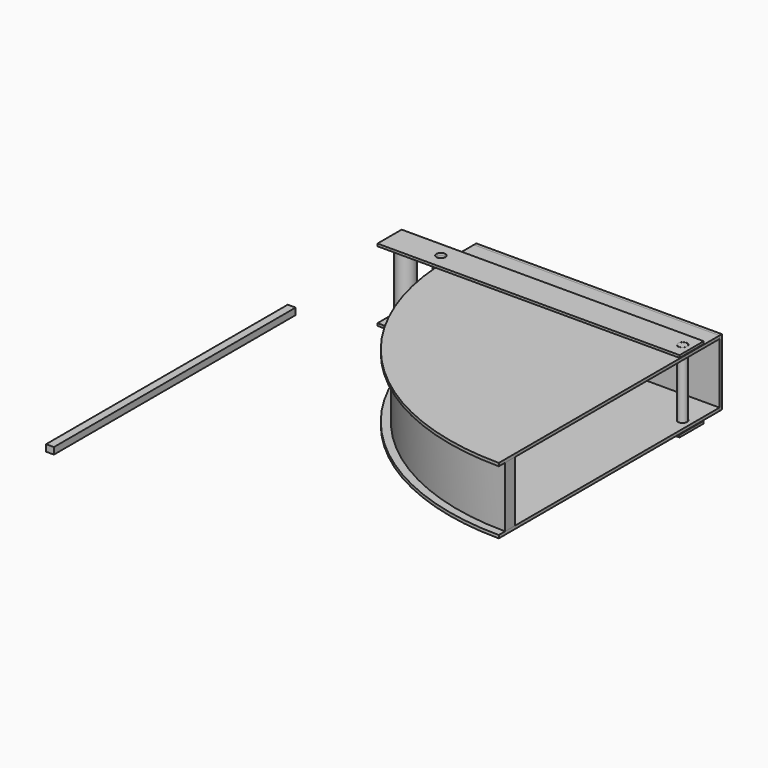
from build123d import *

# Parameters (mm, degrees)
F1_DEPTH  = 100
F4_DEPTH  = 5
F6_W      = 393.5
F6_H      = 50
F6_W_2    = 13
F7_DEPTH  = 5
F9_W      = 406.5
F9_H      = 110
F10_DEPTH = 5.1
F11_R     = 7.5
F12_DEPTH = 110.001
F14_R     = 7.25
F15_DEPTH = 120
F17_W     = 500
F17_H     = 50
F17_R     = 7.5
F18_DEPTH = 4
F0_W      = 20
F0_H      = 50
F21_DEPTH = 100
F22_R     = 15
F23_DEPTH = 112
F24_R     = 11
F24_R_2   = 7.5
F25_DEPTH = 112
F26_W     = 13
F26_H     = 500
F27_DEPTH = 11


# Not quite as in the source:
# - a feature names something its author has since deleted; it is built from what else it names


with BuildPart() as f1:
    # F0 (on Top) → F1 (new body)
    with BuildSketch(Plane.XY):
        with BuildLine():
            ThreePointArc((0, -373.5), (-264.1043827732, -264.1043827732), (-373.5, 0))
            Line((-373.5, 0), (-393.5, 0))
            ThreePointArc((-393.5, 0), (-278.2465183969, -278.2465183969), (0, -393.5))
            Line((0, -393.5), (0, -373.5))
        make_face()
    extrude(amount=F1_DEPTH)


with BuildPart() as f4:
    # F3 (on offset) → F4 (new body)
    with BuildSketch(Plane(origin=(0, 0, 0), x_dir=(1, 0, 0), z_dir=(0, 0, -1))):
        with BuildLine():
            Line((-393.5, 0), (0, 0))
            Line((0, 0), (0, 393.5))
            ThreePointArc((0, 393.5), (-278.2465183969, 278.2465183969), (-393.5, 0))
        make_face()
        Polygon((0, -50), (0, 0), (-393.5, 0), (-406.5, 0), (-406.5, -50), align=None)
        with BuildLine():
            ThreePointArc((-393.5, 0), (-278.2465183969, 278.2465183969), (0, 393.5))
            Line((0, 393.5), (0, 406.5))
            ThreePointArc((0, 406.5), (-287.4389065523, 287.4389065523), (-406.5, 0))
            Line((-406.5, 0), (-393.5, 0))
        make_face()
    extrude(amount=F4_DEPTH)


with BuildPart() as f7:
    # F6 (on offset) → F7 (new body)
    with BuildSketch(Plane.XY.offset(100)):
        with BuildLine():
            Line((0, -393.5), (0, 0))
            Line((0, 0), (-393.5, 0))
            ThreePointArc((-393.5, 0), (-278.2465183969, -278.2465183969), (0, -393.5))
        make_face()
        with Locations((-196.75, 25)):
            Rectangle(F6_W, F6_H)
        with BuildLine():
            Line((0, -406.5), (0, -393.5))
            ThreePointArc((0, -393.5), (-278.2465183969, -278.2465183969), (-393.5, 0))
            Line((-393.5, 0), (-406.5, 0))
            ThreePointArc((-406.5, 0), (-287.4389065523, -287.4389065523), (0, -406.5))
        make_face()
        with Locations((-400, 25)):
            Rectangle(F6_W_2, F6_H)
    extrude(amount=F7_DEPTH)


with BuildPart() as f10:
    # F9 (on offset) → F10 (new body)
    with BuildSketch(Plane(origin=(0, 50, 0), x_dir=(-1, 0, 0), z_dir=(0, 1, 0))):
        with Locations((203.25, 50)):
            Rectangle(F9_W, F9_H)
    extrude(amount=F10_DEPTH)


with BuildPart() as f12_tool:
    # F11 (on face) → F12 (new body, through all)
    with BuildSketch(Plane.XY.offset(105)):
        with Locations((-15, -7.5)):
            Circle(F11_R)
    extrude(amount=-F12_DEPTH)


with BuildPart() as f4_1:
    add(f4.part)

    # F12: cut by f12_tool
    add(f12_tool.part, mode=Mode.SUBTRACT)


with BuildPart() as f7_1:
    add(f7.part)

    # F12: cut by f12_tool
    add(f12_tool.part, mode=Mode.SUBTRACT)


with BuildPart() as f15:
    # F14 (on offset) → F15 (new body)
    with BuildSketch(Plane.XY.offset(110)):
        with Locations((-15, -7.5)):
            Circle(F14_R)
    extrude(amount=-F15_DEPTH)


with BuildPart() as f18:
    # F17 (on offset) → F18 (new body)
    with BuildSketch(Plane.XY.offset(110)):
        with Locations((-250, -7.5)):
            Rectangle(F17_W, F17_H)
        with Locations((-415, -7.5)):
            Circle(F17_R, mode=Mode.SUBTRACT)
        with Locations((-15, -7.5)):
            Circle(F17_R, mode=Mode.SUBTRACT)
    extrude(amount=-F18_DEPTH)


with BuildPart() as f20_1:
    # F20: instance of F18
    add(f18.part.mirror(Plane(origin=(-244.1990168857, -244.1990168857, 50), x_dir=(1, 0, 0), z_dir=(0, 0, 1))))


with BuildPart() as f21:
    # F0 (on Top) → F21 (new body)
    with BuildSketch(Plane.XY):
        with Locations((-383.5, 25)):
            Rectangle(F0_W, F0_H)
    extrude(amount=F21_DEPTH)


with BuildPart() as f23:
    # F22 (on face) → F23 (new body, through all)
    with BuildSketch(Plane.XY.offset(-6)):
        with Locations((-473.5828638077, -7.5)):
            Circle(F22_R)
    extrude(amount=F23_DEPTH)


with BuildPart() as f25:
    # F24 (on face) → F25 (new body, through all)
    with BuildSketch(Plane(origin=(0, 0, 106), x_dir=(1, 0, 0), z_dir=(0, 0, -1))):
        with Locations((-415, 7.5)):
            Circle(F24_R)
        with Locations((-415, 7.5)):
            Circle(F24_R_2, mode=Mode.SUBTRACT)
    extrude(amount=F25_DEPTH)


with BuildPart() as f27:
    # F26 (on Top) → F27 (new body)
    with BuildSketch(Plane.XY):
        with Locations((-595.9782657623, -340.0288820267)):
            Rectangle(F26_W, F26_H)
    extrude(amount=F27_DEPTH)


solid = Compound([f1.part, f10.part, f4_1.part, f7_1.part, f15.part, f18.part, f20_1.part, f21.part, f23.part, f25.part, f27.part])
